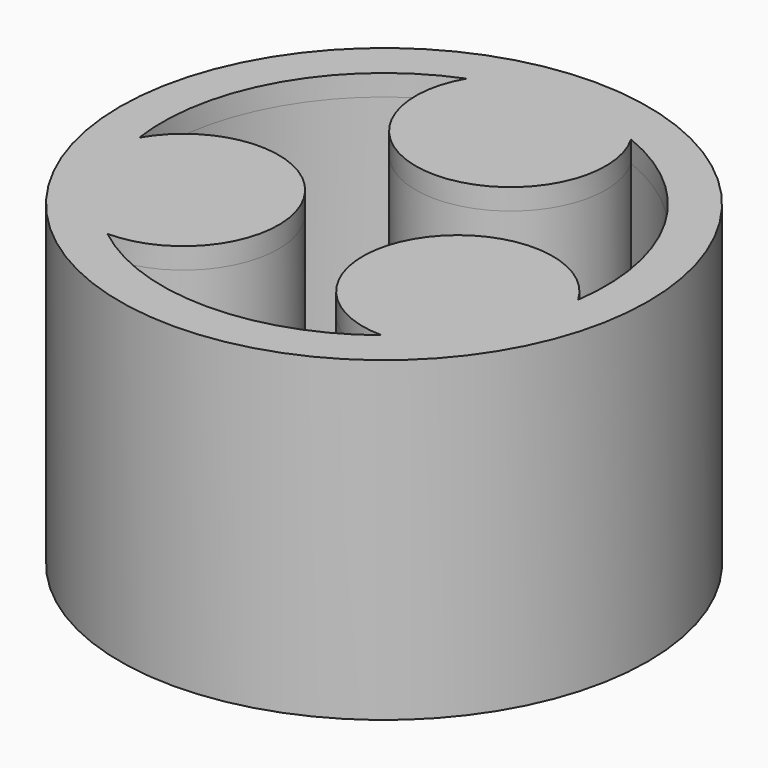
from build123d import *

# Parameters (mm, degrees)
F0_R     = 25
F0_R_2   = 5
F0_R_3   = 3
F0_R_4   = 3.5
F1_DEPTH = 28
F2_T     = -4
F3_DEPTH = 25
F4_R     = 25
F5_DEPTH = 2


# Not quite as in the source:
# - a feature names something its author has since deleted; it is built from what else it names


with BuildPart() as f1:
    # F0 (on Top) → F1 (new body)
    with BuildSketch(Plane.XY):
        Circle(F0_R)
        with Locations((-12.990381, -7.5)):
            Circle(F0_R_2, mode=Mode.SUBTRACT)
        with Locations((0, -15)):
            Circle(F0_R_3, mode=Mode.SUBTRACT)
        with Locations((12.990381, -7.5)):
            Circle(F0_R_2, mode=Mode.SUBTRACT)
        with Locations((-12.990381, 7.5)):
            Circle(F0_R_3, mode=Mode.SUBTRACT)
        Circle(F0_R_4, mode=Mode.SUBTRACT)
        with Locations((12.990381, 7.5)):
            Circle(F0_R_3, mode=Mode.SUBTRACT)
        with Locations((0, 15)):
            Circle(F0_R_2, mode=Mode.SUBTRACT)
        Circle(F0_R_4)
        with Locations((-12.990381, 7.5)):
            Circle(F0_R_3)
        with Locations((12.990381, 7.5)):
            Circle(F0_R_3)
        with Locations((0, -15)):
            Circle(F0_R_3)
    extrude(amount=F1_DEPTH)

    # F2
    f2_openings = [f1.faces().sort_by_distance(p)[0] for p in [
        (0, 0, 28),
    ]]
    offset(amount=F2_T, openings=f2_openings)

    # F0 (on Top) → F3 (cut)
    with BuildSketch(Plane.XY):
        with Locations((-12.990381, 7.5)):
            Circle(F0_R_3)
        Circle(F0_R_4)
        with Locations((12.990381, 7.5)):
            Circle(F0_R_3)
        with Locations((0, -15)):
            Circle(F0_R_3)
    extrude(amount=F3_DEPTH, mode=Mode.SUBTRACT)

    # F4 (on face) → F5 (join)
    with BuildSketch(Plane.XY.offset(28)):
        Circle(F4_R)
        with BuildLine():
            ThreePointArc((-20.78461, -3), (-18.186533, 10.5), (-7.794229, 19.5))
            ThreePointArc((-7.794229, 19.5), (0, 6), (7.794229, 19.5))
            ThreePointArc((7.794229, 19.5), (18.186533, 10.5), (20.78461, -3))
            ThreePointArc((20.78461, -3), (5.196152, -3), (12.990381, -16.5))
            ThreePointArc((12.990381, -16.5), (0, -21), (-12.990381, -16.5))
            ThreePointArc((-12.990381, -16.5), (-5.196152, -3), (-20.78461, -3))
        make_face(mode=Mode.SUBTRACT)
    extrude(amount=F5_DEPTH)


solid = f1.part
